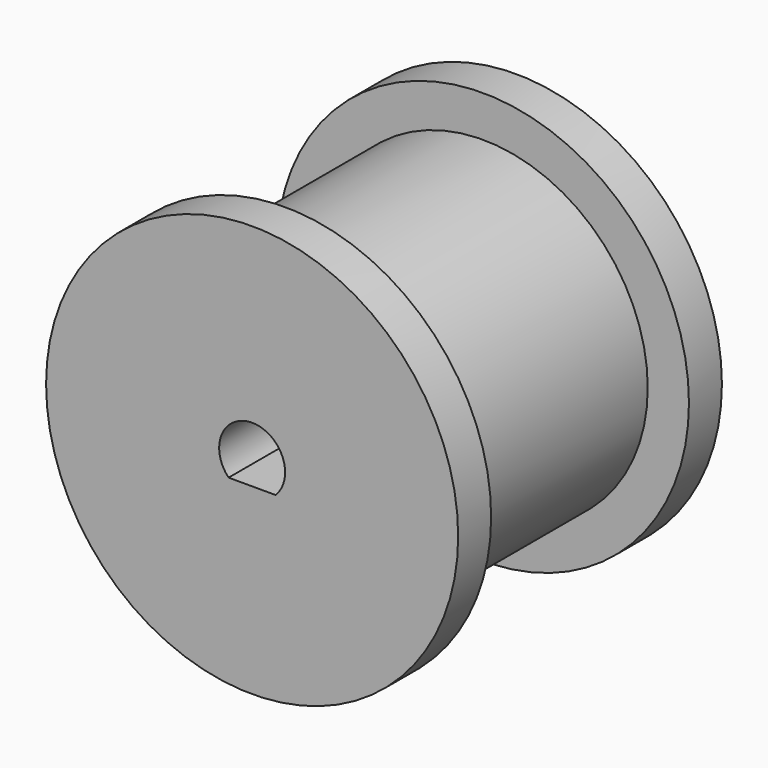
from build123d import *

# Parameters (mm, degrees)
F0_R     = 12.7
F1_DEPTH = 25.4
F2_R     = 15.875
F2_R_2   = 12.7
F3_DEPTH = 3.175


with BuildPart() as f1:
    # F0 (on Front) → F1 (new body)
    with BuildSketch(Plane.XZ):
        Circle(F0_R)
        with BuildLine():
            ThreePointArc((-1.8139228208, -1.778), (-0.9602697629, 2.351485059), (2.54, 0))
            ThreePointArc((2.54, 0), (2.351485059, -0.9602697629), (1.8139228208, -1.778))
            ThreePointArc((1.8139228208, -1.778), (0, -2.54), (-1.8139228208, -1.778))
        make_face(mode=Mode.SUBTRACT)
        with BuildLine():
            Line((1.8139228208, -1.778), (-1.8139228208, -1.778))
            ThreePointArc((-1.8139228208, -1.778), (0, -2.54), (1.8139228208, -1.778))
        make_face()
    extrude(amount=F1_DEPTH)

    # F2 (on face) → F3 (join)
    with BuildSketch(Plane.XZ.offset(25.4)):
        Circle(F2_R)
        Circle(F2_R_2, mode=Mode.SUBTRACT)
    extrude(amount=-F3_DEPTH)

    # F5: F1 across plane


with BuildPart() as f1_1:
    add(f1.part)
    add(f1.part.mirror(Plane(origin=(0, -12.7, -0.0066463366), x_dir=(1, 0, 0), z_dir=(0, 1, 0))))


solid = f1_1.part
